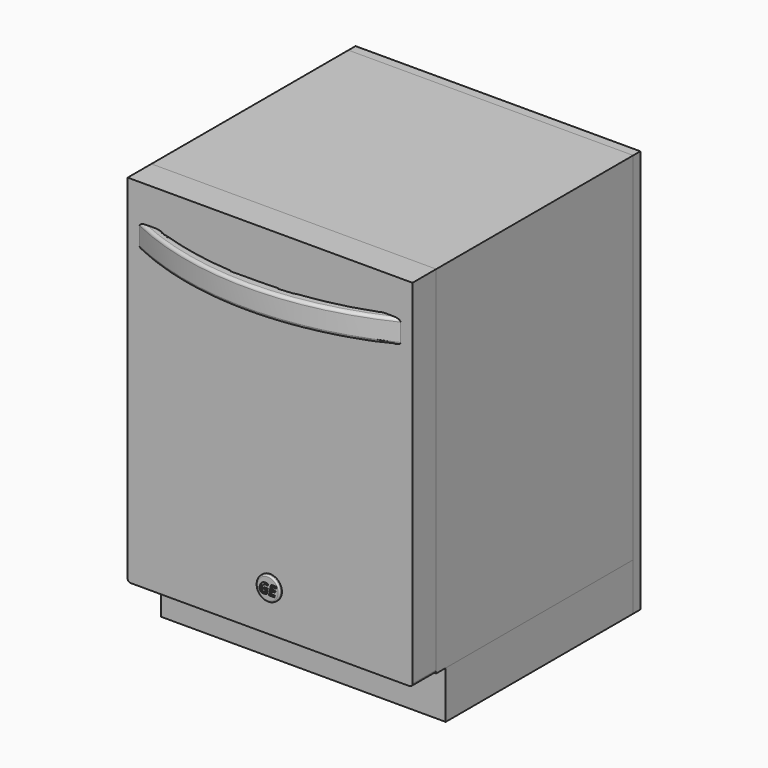
from build123d import *

# Parameters (mm, degrees)
F0_W          = 609.6
F0_H          = 762
F0_R          = 25.4
F0_W_2        = 558.8
F0_H_2        = 50.8
F1_DEPTH      = 63.5
F0_H_3        = 101.6
F2_DEPTH      = 527.05
F3_DEPTH      = 127
F4_W          = 457.2
F4_H          = 38.1
F5_DEPTH      = 787.401
F6_T1_DEPTH   = 50.8
F6_T3_DEPTH   = 50.8
F6_T5_DEPTH   = 1447.8
F6_T7_DEPTH   = 1447.8
F7_R          = 6.35
F8_DEPTH      = 527.05
F9_R          = 6.35
F10_DEPTH     = 69.85
F11_R         = 3.175
F12_TEXT_SIZE = 30.0888450148
F13_DEPTH     = 3.175
F14_DEPTH     = 25.4
F15_W         = 609.6
F15_H         = 863.6
F16_DEPTH     = 19.05


# Not quite as in the source:
# - a fillet or chamfer that OpenCascade refuses, or shapes differently, is made with other operations: its cross-section is extruded or revolved along the edge and cut away or added
# - Text() gives the source's letters only with a copy of the font that has no kerning and outlines rounded to 1/6400 em; it was checked with that copy


with BuildPart() as f1:
    # F0 (on Front) → F1 (new body)
    with BuildSketch(Plane.XZ):
        with Locations((0, 50.8)):
            Rectangle(F0_W, F0_H)
        with Locations((0, -241.3)):
            Circle(F0_R, mode=Mode.SUBTRACT)
        with Locations((0, 330.2)):
            Rectangle(F0_W_2, F0_H_2, mode=Mode.SUBTRACT)
        with Locations((0, 330.2)):
            Rectangle(F0_W_2, F0_H_2)
        with Locations((0, -241.3)):
            Circle(F0_R)
    extrude(amount=F1_DEPTH)

    # F0 (on Front) → F3 (join)
    with BuildSketch(Plane.XZ):
        with Locations((0, 330.2)):
            Rectangle(F0_W_2, F0_H_2)
    extrude(amount=F3_DEPTH)

    # F4 (on face) → F5 (cut, through all)
    with BuildSketch(Plane.XY.offset(355.6)):
        with Locations((0, -82.55)):
            Rectangle(F4_W, F4_H)
    extrude(amount=-F5_DEPTH, mode=Mode.SUBTRACT)

    # F6: fillet of radius 646.43 on 4 edges, made by hand

    # F6_s2 → F6_t1 (join)
    with BuildSketch(Plane.XY.offset(304.8)):
        with BuildLine():
            ThreePointArc((-228.6, -63.5), (-120.9240321185, -92.0037721886), (-9.9533535588, -101.6))
            Line((-9.9533535588, -101.6), (-228.6, -101.6))
            Line((-228.6, -101.6), (-228.6, -63.5))
        make_face()
    extrude(amount=F6_T1_DEPTH)

    # F6_s4 → F6_t3 (join)
    with BuildSketch(Plane.XY.offset(304.8)):
        with BuildLine():
            ThreePointArc((228.6, -63.5), (120.9240321185, -92.0037721886), (9.9533535588, -101.6))
            Line((9.9533535588, -101.6), (228.6, -101.6))
            Line((228.6, -101.6), (228.6, -63.5))
        make_face()
    extrude(amount=F6_T3_DEPTH)

    # F6_s6 → F6_t5 (cut)
    with BuildSketch(Plane.XY.offset(-393.7)):
        with BuildLine():
            ThreePointArc((-279.4, -63.5), (-143.262529993, -110.9251319693), (0, -127))
            Line((0, -127), (-279.4, -127))
            Line((-279.4, -127), (-279.4, -63.5))
        make_face()
    extrude(amount=F6_T5_DEPTH, mode=Mode.SUBTRACT)

    # F6_s8 → F6_t7 (cut)
    with BuildSketch(Plane.XY.offset(-393.7)):
        with BuildLine():
            ThreePointArc((279.4, -63.5), (143.262529993, -110.9251319693), (0, -127))
            Line((0, -127), (279.4, -127))
            Line((279.4, -127), (279.4, -63.5))
        make_face()
    extrude(amount=F6_T7_DEPTH, mode=Mode.SUBTRACT)

    # F7
    f7_edges = [f1.edges().sort_by_distance(p)[0] for p in [
        (0, -127, 355.6),
        (0, -101.6, 355.6),
        (0, -127, 304.8),
        (0, -101.6, 304.8),
    ]]
    fillet(f7_edges, radius=F7_R)


with BuildPart() as f2:
    # F0 (on Front) → F2 (new body)
    with BuildSketch(Plane.XZ):
        with Locations((0, -381)):
            Rectangle(F0_W, F0_H_3)
    extrude(amount=-F2_DEPTH)

    # F14 (cut): a face of the model
    f14_faces = [f2.faces().sort_by_distance(p)[0] for p in [
        (0, 0, -381),
    ]]
    extrude(f14_faces, amount=-F14_DEPTH, mode=Mode.SUBTRACT)


with BuildPart() as f8:
    # F8 (new, through all): a face of the model
    f8_faces = [f1.part.faces().sort_by_distance(p)[0] for p in [
        (0, 0, 50.8),
    ]]
    extrude(f8_faces, amount=F8_DEPTH)


with BuildPart() as f1_1:
    add(f1.part)

    # F9
    f9_edges = [f1_1.edges().sort_by_distance(p)[0] for p in [
        (-304.8, -31.75, -330.2),
        (304.8, -31.75, -330.2),
    ]]
    fillet(f9_edges, radius=F9_R)


with BuildPart() as f10:
    # F0 (on Front) → F10 (new body)
    with BuildSketch(Plane.XZ):
        with Locations((0, -241.3)):
            Circle(F0_R)
    extrude(amount=F10_DEPTH)

    # F11
    f11_edges = [f10.edges().sort_by_distance(p)[0] for p in [
        (-25.4, -69.85, -241.3),
    ]]
    fillet(f11_edges, radius=F11_R)

    # F12 (on face) → F13 (cut)
    with BuildSketch(Plane.XZ.offset(69.85)):
        with Locations((-19.1044491183, -252.8377498543)):
            Text('GE', F12_TEXT_SIZE, font='Open Sans', font_style=FontStyle.BOLDITALIC, text_align=(TextAlign.LEFT, TextAlign.BOTTOM))
    extrude(amount=-F13_DEPTH, mode=Mode.SUBTRACT)


with BuildPart() as f16:
    # F15 (on face) → F16 (new body)
    with BuildSketch(Plane(origin=(0, 527.05, 0), x_dir=(-1, 0, 0), z_dir=(0, 1, 0))):
        Rectangle(F15_W, F15_H)
    extrude(amount=F16_DEPTH)


solid = Compound([f2.part, f8.part, f1_1.part, f10.part, f16.part])
